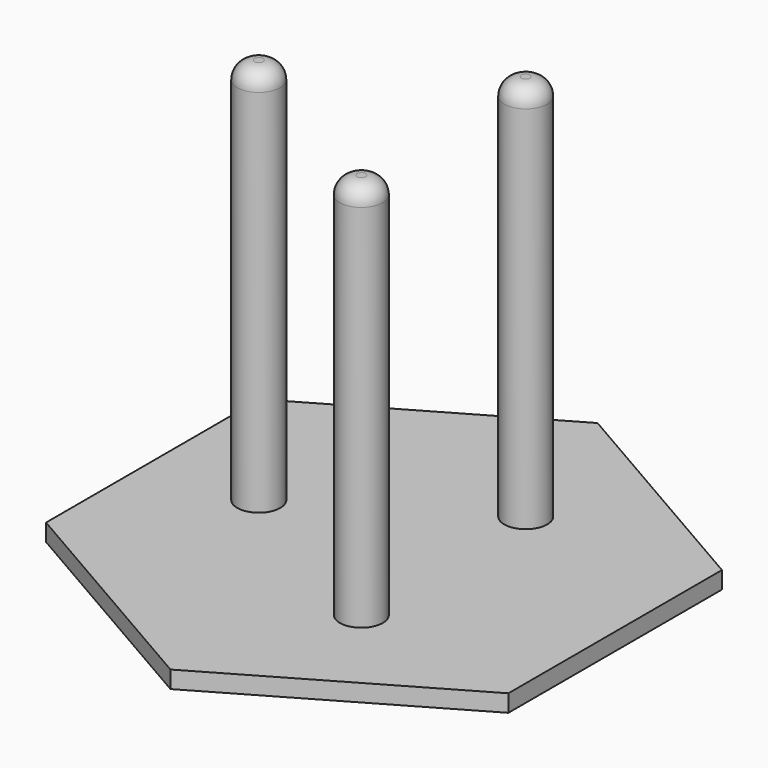
from build123d import *

# Parameters (mm, degrees)
F0_R     = 22.365
F1_DEPTH = 2
F2_R     = 2.5
F3_DEPTH = 45
F4_R     = 2


# Not quite as in the source:
# - a feature of the source that left no trace in its solid (it failed there, or was rolled back) is left out


with BuildPart() as f1:
    # F0 (on Top) → F1 (new body)
    with BuildSketch(Plane.XY):
        Polygon((26.865, -15.5105149818), (26.865, 15.5105149818), (0, 31.0210299636), (-26.865, 15.5105149818), (-26.865, -15.5105149818), (0, -31.0210299636), align=None)
        Circle(F0_R, mode=Mode.SUBTRACT)
        Circle(F0_R)
    extrude(amount=F1_DEPTH)

    # F2 (on face) → F3 (join)
    with BuildSketch(Plane.XY.offset(2)):
        with Locations((-14.5547939909, 0)):
            Circle(F2_R)
        with Locations((6.3876030045, 12.604821343)):
            Circle(F2_R)
        with Locations((6.8325, -11.8342371427)):
            Circle(F2_R)
    extrude(amount=F3_DEPTH)

    # F4
    f4_edges = [f1.edges().sort_by_distance(p)[0] for p in [
        (-17.054794, 0, 47),
        (4.3325, -11.834237, 47),
        (3.887603, 12.604821, 47),
    ]]
    fillet(f4_edges, radius=F4_R)


solid = f1.part
